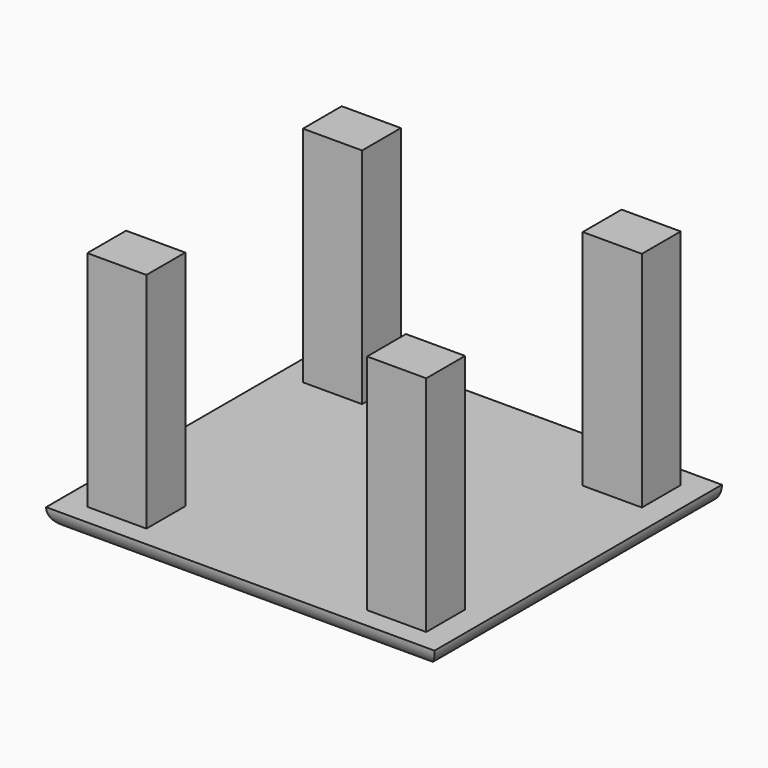
from build123d import *

# Parameters (mm, degrees)
F0_W     = 6.0909511521
F0_H     = 5
F0_H_2   = 2.6896382868
F0_H_3   = 2.3103617132
F1_DEPTH = 2
F2_DEPTH = 25
F4_R     = 1.99999
F5_R     = 6.305532295
F6_DEPTH = 76


# Not quite as in the source:
# - a fillet or chamfer is up to 0.001 mm smaller than in the source, because OpenCascade refuses the exact size
# - an extrude ends at something that could not be found from the text; its depth is read off the source's solid


with BuildPart() as f1:
    # F0 (on Top) → F1 (new body)
    with BuildSketch(Plane.XY):
        Polygon((-17.4544863403, 13.6900003999), (-20, 13.6900003999), (-20, -18.5), (20, -18.5), (20, 13.6900003999), (17.4544863403, 13.6900003999), (17.4544863403, 11.3796386868), (11.3635351881, 11.3796386868), (11.3635351881, 13.6900003999), (-11.3635351881, 13.6900003999), (-11.3635351881, 11.3796386868), (-17.4544863403, 11.3796386868), align=None)
        with Locations((-14.4090107642, -13.8796386868)):
            Rectangle(F0_W, F0_H, mode=Mode.SUBTRACT)
        with Locations((14.4090107642, -13.8796386868)):
            Rectangle(F0_W, F0_H, mode=Mode.SUBTRACT)
        Polygon((20, 18.5), (-20, 18.5), (-20, 13.6900003999), (-17.4544863403, 13.6900003999), (-17.4544863403, 16.3796386868), (-11.3635351881, 16.3796386868), (-11.3635351881, 13.6900003999), (11.3635351881, 13.6900003999), (11.3635351881, 16.3796386868), (17.4544863403, 16.3796386868), (17.4544863403, 13.6900003999), (20, 13.6900003999), align=None)
        with Locations((14.4090107642, -13.8796386868)):
            Rectangle(F0_W, F0_H)
        with Locations((-14.4090107642, -13.8796386868)):
            Rectangle(F0_W, F0_H)
        with Locations((-14.4090107642, 15.0348195434)):
            Rectangle(F0_W, F0_H_2)
        with Locations((14.4090107642, 15.0348195434)):
            Rectangle(F0_W, F0_H_2)
        with Locations((14.4090107642, 12.5348195434)):
            Rectangle(F0_W, F0_H_3)
        with Locations((-14.4090107642, 12.5348195434)):
            Rectangle(F0_W, F0_H_3)
    extrude(amount=F1_DEPTH)

    # F0 (on Top) → F2 (join)
    with BuildSketch(Plane.XY):
        with Locations((14.4090107642, -13.8796386868)):
            Rectangle(F0_W, F0_H)
        with Locations((14.4090107642, 12.5348195434)):
            Rectangle(F0_W, F0_H_3)
        with Locations((14.4090107642, 15.0348195434)):
            Rectangle(F0_W, F0_H_2)
        with Locations((-14.4090107642, 12.5348195434)):
            Rectangle(F0_W, F0_H_3)
        with Locations((-14.4090107642, 15.0348195434)):
            Rectangle(F0_W, F0_H_2)
        with Locations((-14.4090107642, -13.8796386868)):
            Rectangle(F0_W, F0_H)
    extrude(amount=F2_DEPTH)

    # F4 (radius 2 in the source; OpenCascade refuses exactly that, so slightly less here)
    f4_edges = [f1.edges().sort_by_distance(p)[0] for p in [
        (20, 0, 0),
        (-20, 0, 0),
        (0, -18.5, 0),
    ]]
    fillet(f4_edges, radius=F4_R)

    # F5 (on face) → F6 (cut, through all)
    with BuildSketch(Plane(origin=(0, 13.6900003999, 0), x_dir=(-1, 0, 0), z_dir=(0, 1, 0))):
        with Locations((0, -14.4779002294)):
            Circle(F5_R)
    extrude(amount=F6_DEPTH, mode=Mode.SUBTRACT)


solid = f1.part
